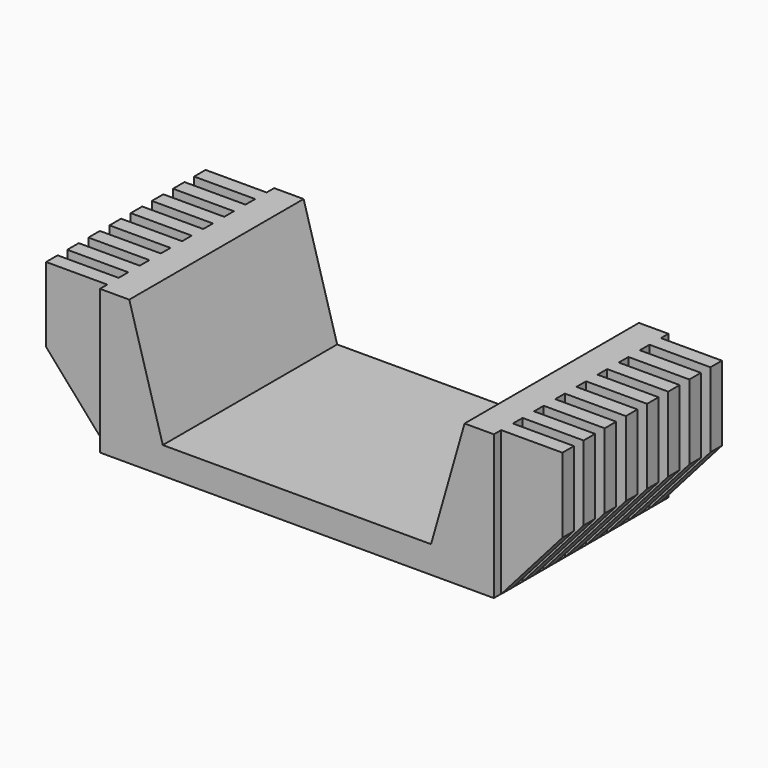
from build123d import *

# Parameters (mm, degrees)
F0_W     = 39.116
F0_H     = 16.51
F1_DEPTH = 10.922
F2_W     = 4.6228
F2_H     = 0.7122
F2_W_2   = 4.6149979224
F2_H_2   = 0.9144
F2_W_3   = 4.6228001026
F2_W_4   = 4.6377839463
F2_H_3   = 0.6950350265
F3_DEPTH = 10.923
F5_DEPTH = 16.511
F7_DEPTH = 16.511


# Not quite as in the source:
# - a feature names something its author has since deleted; it is built from what else it names


with BuildPart() as f1:
    # F0 (on Top) → F1 (new body)
    with BuildSketch(Plane.XY):
        Rectangle(F0_W, F0_H)
    extrude(amount=F1_DEPTH)

    # F2 (on face) → F3 (cut, through all)
    with BuildSketch(Plane.XY.offset(10.922)):
        with Locations((-17.2466, 7.8989)):
            Rectangle(F2_W, F2_H)
        Polygon((-14.9352, 6.462406421), (-19.558, 6.4552534719), (-19.558, 5.548006421), (-14.9352, 5.548006421), align=None)
        with Locations((-17.2505010388, 4)):
            Rectangle(F2_W_2, F2_H_2)
        with Locations((-17.2466, 2)):
            Rectangle(F2_W, F2_H_2)
        with Locations((-17.2466, 0)):
            Rectangle(F2_W, F2_H_2)
        with Locations((-17.2466, -2.0119585525)):
            Rectangle(F2_W, F2_H_2)
        with Locations((-17.2465999487, -4.0119585525)):
            Rectangle(F2_W_3, F2_H_2)
        with Locations((-17.2465999487, -6.0119585525)):
            Rectangle(F2_W_3, F2_H_2)
        Polygon((-14.9202160537, -8.4639521315), (-14.9202160537, -8.255), (-19.558, -8.255), (-19.558, -7.5599649735), (-21.6498160537, -7.5599649735), (-21.6498160537, -8.4639521315), align=None)
        with Locations((-17.2391080269, -7.9074824868)):
            Rectangle(F2_W_4, F2_H_3)
        Polygon((21.6498160537, -7.5599649735), (19.558, -7.5599649735), (19.558, -8.255), (14.9202160537, -8.255), (14.9202160537, -8.4639521315), (21.6498160537, -8.4639521315), align=None)
        with Locations((17.2391080269, -7.9074824868)):
            Rectangle(F2_W_4, F2_H_3)
        with Locations((17.2465999487, -6.0119585525)):
            Rectangle(F2_W_3, F2_H_2)
        with Locations((17.2465999487, -4.0119585525)):
            Rectangle(F2_W_3, F2_H_2)
        with Locations((17.2466, -2.0119585525)):
            Rectangle(F2_W, F2_H_2)
        with Locations((17.2466, 0)):
            Rectangle(F2_W, F2_H_2)
        with Locations((17.2466, 2)):
            Rectangle(F2_W, F2_H_2)
        with Locations((17.2505010388, 4)):
            Rectangle(F2_W_2, F2_H_2)
        Polygon((14.9352, 5.548006421), (19.558, 5.548006421), (19.558, 6.4552534719), (14.9352, 6.462406421), align=None)
        with Locations((17.2466, 7.8989)):
            Rectangle(F2_W, F2_H)
    extrude(amount=-F3_DEPTH, mode=Mode.SUBTRACT)

    # F4 (on face) → F5 (cut, through all)
    with BuildSketch(Plane.XZ.offset(8.255)):
        Polygon((12.7, 10.922), (-12.7, 10.922), (-10.16, 2.0491317846), (0, 2.0491317846), (10.16, 2.0491317846), align=None)
    extrude(amount=-F5_DEPTH, mode=Mode.SUBTRACT)

    # F6 (on face) → F7 (cut, through all)
    with BuildSketch(Plane(origin=(0, 8.255, 0), x_dir=(-1, 0, 0), z_dir=(0, 1, 0))):
        Polygon((-20.5232, 0), (-14.9352, 0), (-20.5232, 6.35), align=None)
        Polygon((20.5232, 6.35), (14.9352, 0), (20.5232, 0), align=None)
    extrude(amount=-F7_DEPTH, mode=Mode.SUBTRACT)


solid = f1.part
